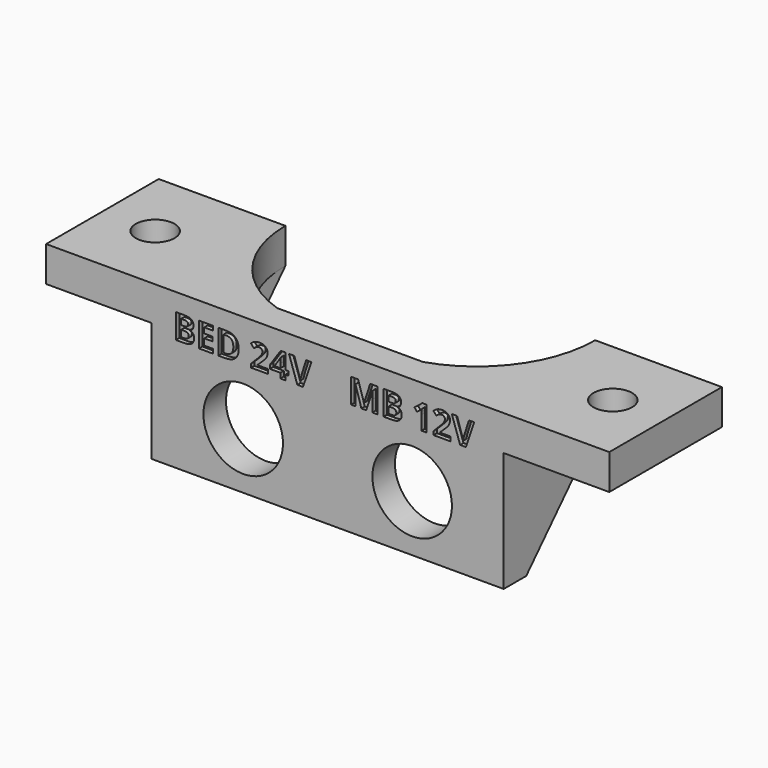
from build123d import *

# Parameters (mm, degrees)
F0_W         = 50
F0_H         = 22
F0_R         = 5.65
F2_DEPTH     = 4
F3_R         = 2.75
F3_W         = 3
F3_H         = 16
F4_DEPTH     = 5
F5_DEPTH     = 22
F7_DEPTH     = 65.001
F1_TEXT_SIZE = 4.8920313396
F8_DEPTH     = 0.6


# Not quite as in the source:
# - Text() gives the source's letters only with a copy of the font that has no kerning and outlines rounded to 1/6400 em; it was checked with that copy


with BuildPart() as f2:
    # F0 (on Front) → F2 (new body)
    with BuildSketch(Plane.XZ):
        Rectangle(F0_W, F0_H)
        with Locations((-12, -3)):
            Circle(F0_R, mode=Mode.SUBTRACT)
        with Locations((12, -3)):
            Circle(F0_R, mode=Mode.SUBTRACT)
    extrude(amount=-F2_DEPTH)

    # F3 (on face) → F4 (join)
    with BuildSketch(Plane.XY.offset(11)):
        Polygon((-40, 20), (-40, 0), (-25, 0), (-25, 4), (-25, 20), align=None)
        with Locations((-32.5, 10)):
            Circle(F3_R, mode=Mode.SUBTRACT)
        Polygon((25, 4), (25, 0), (40, 0), (40, 20), (25, 20), align=None)
        with Locations((32.5, 10)):
            Circle(F3_R, mode=Mode.SUBTRACT)
        with Locations((-23.5, 12)):
            Rectangle(F3_W, F3_H)
        with Locations((23.5, 12)):
            Rectangle(F3_W, F3_H)
        with BuildLine():
            Line((-22, 20), (-22, 4))
            Line((-22, 4), (-10.3636363636, 4))
            ThreePointArc((-10.3636363636, 4), (-18.7832886906, 10.1080214482), (-22, 20))
        make_face()
        with BuildLine():
            Line((10.3636363636, 4), (22, 4))
            Line((22, 4), (22, 20))
            ThreePointArc((22, 20), (18.7832886906, 10.1080214482), (10.3636363636, 4))
        make_face()
    extrude(amount=-F4_DEPTH)

    # F3 (on face) → F5 (join, through all)
    with BuildSketch(Plane.XY.offset(11)):
        with Locations((-23.5, 12)):
            Rectangle(F3_W, F3_H)
        with Locations((23.5, 12)):
            Rectangle(F3_W, F3_H)
    extrude(amount=-F5_DEPTH)

    # F6 (on face) → F7 (cut, through all)
    with BuildSketch(Plane(origin=(-25, 0, 0), x_dir=(0, -1, 0), z_dir=(-1, 0, 0))):
        Polygon((-4, -11), (-20, 6), (-20, -11), align=None)
    extrude(amount=-F7_DEPTH, mode=Mode.SUBTRACT)

    # F1 (on Front) → F8 (cut)
    with BuildSketch(Plane.XZ):
        with Locations((-22, 5)):
            Text('BED 24V', F1_TEXT_SIZE, font='Open Sans', font_style=FontStyle.BOLD, text_align=(TextAlign.LEFT, TextAlign.BOTTOM))
        with Locations((2.8744506019, 5)):
            Text('MB 12V', F1_TEXT_SIZE, font='Open Sans', font_style=FontStyle.BOLD, text_align=(TextAlign.LEFT, TextAlign.BOTTOM))
    extrude(amount=-F8_DEPTH, mode=Mode.SUBTRACT)


solid = f2.part
